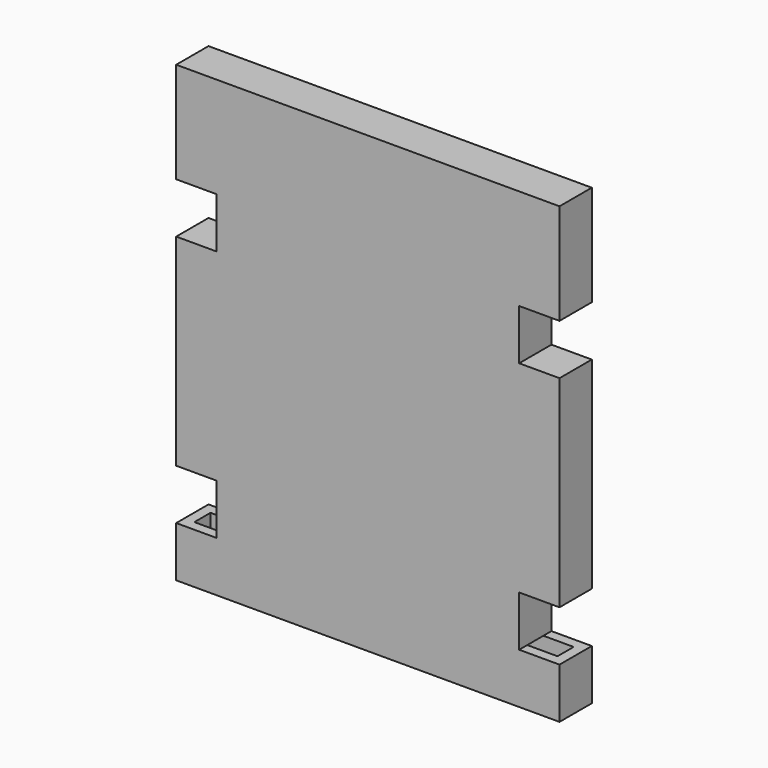
from build123d import *

# Parameters (mm, degrees)
F0_W     = 10.16
F0_H     = 12.7
F0_H_2   = 50.8
F0_H_3   = 25.4
F1_DEPTH = 5.08
F2_T     = -2.54


# Not quite as in the source:
# - a shell that OpenCascade refuses in one call is made with other operations: the cavity is built on its own and cut out


with BuildPart() as f1:
    # F0 (on Front) → F1 (new body, symmetric)
    with BuildSketch(Plane.XZ):
        Polygon((-38.1, -57.15), (38.1, -57.15), (38.1, -44.45), (38.1, -31.75), (38.1, 19.05), (38.1, 31.75), (38.1, 57.15), (-38.1, 57.15), (-38.1, 31.75), (-38.1, 19.05), (-38.1, -31.75), (-38.1, -44.45), align=None)
        with Locations((43.18, -50.8)):
            Rectangle(F0_W, F0_H)
        with Locations((-43.18, -50.8)):
            Rectangle(F0_W, F0_H)
        with Locations((43.18, -6.35)):
            Rectangle(F0_W, F0_H_2)
        with Locations((-43.18, -6.35)):
            Rectangle(F0_W, F0_H_2)
        with Locations((43.18, 44.45)):
            Rectangle(F0_W, F0_H_3)
        with Locations((-43.18, 44.45)):
            Rectangle(F0_W, F0_H_3)
    extrude(amount=F1_DEPTH, both=True)

    # F2: a shell. OpenCascade refuses it in one call, so the cavity is built on its own and cut out:
    # the body offset inwards by the wall thickness, plus a prism from it out through each open face.
    f2_core = offset(f1.part, amount=F2_T, kind=Kind.INTERSECTION, mode=Mode.PRIVATE)
    f2_exits = [f2_core.faces().sort_by_distance(p)[0] for p in [
        (40.64, 0, 34.29),
        (40.64, 0, -46.99),
        (-40.64, 0, -46.99),
        (-40.64, 0, 34.29),
    ]]
    add(f2_core, mode=Mode.SUBTRACT)
    extrude(f2_exits, amount=-F2_T, mode=Mode.SUBTRACT)


solid = f1.part
